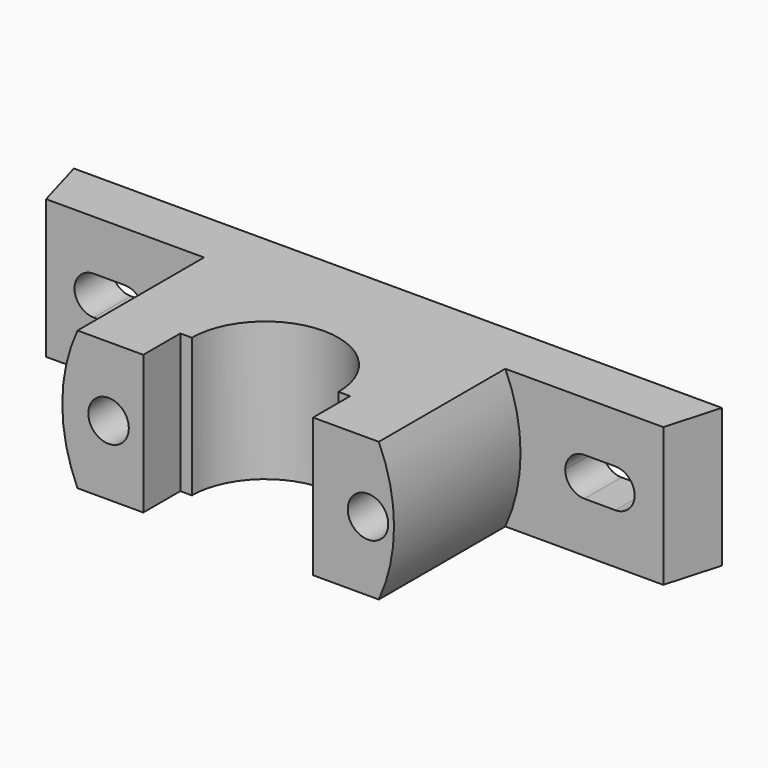
from build123d import *

# Parameters (mm, degrees)
F0_W         = 168
F0_H         = 36
F1_DEPTH     = 14
F3_DEPTH     = 36.001
F5_DEPTH     = 41
F6_R         = 5.25
F7_DEPTH     = 55.001
F8_W         = 20
F8_H         = 20
F9_DEPTH     = 6.5
F10_W        = 67
F10_H        = 20
F11_DEPTH    = 2
F12_T1_DEPTH = 34.1421356237
F14_DEPTH    = 25
F16_DEPTH    = 36.001


# Not quite as in the source:
# - a fillet or chamfer that OpenCascade refuses, or shapes differently, is made with other operations: its cross-section is extruded or revolved along the edge and cut away or added


with BuildPart() as f1:
    # F0 (on Front) → F1 (new body)
    with BuildSketch(Plane.XZ):
        Rectangle(F0_W, F0_H)
    extrude(amount=F1_DEPTH)

    # F2 (on face) → F3 (cut, through all)
    with BuildSketch(Plane(origin=(0, 0, -18), x_dir=(1, 0, 0), z_dir=(0, 0, -1))):
        Polygon((-84, 14), (-84, 0), (-80, 14), align=None)
        Polygon((80, 14), (84, 0), (84, 14), align=None)
    extrude(amount=-F3_DEPTH, mode=Mode.SUBTRACT)

    # F4 (on face) → F5 (join)
    with BuildSketch(Plane.XZ.offset(14)):
        with BuildLine():
            ThreePointArc((39.0512483795, -18), (43, 0), (39.0512483795, 18))
            Line((39.0512483795, 18), (-39.0512483795, 18))
            ThreePointArc((-39.0512483795, 18), (-43, 0), (-39.0512483795, -18))
            Line((-39.0512483795, -18), (39.0512483795, -18))
        make_face()
    extrude(amount=F5_DEPTH)

    # F6 (on face) → F7 (cut, through all)
    with BuildSketch(Plane.XZ.offset(55)):
        with Locations((36.25, 0)):
            Circle(F6_R)
        with Locations((-31, 0)):
            Circle(F6_R)
    extrude(amount=-F7_DEPTH, mode=Mode.SUBTRACT)

    # F8 (on face) → F9 (cut)
    with BuildSketch(Plane(origin=(0, 0, 0), x_dir=(-1, 0, 0), z_dir=(0, 1, 0))):
        with Locations((-36.25, 0)):
            Rectangle(F8_W, F8_H)
        with Locations((31, 0)):
            Rectangle(F8_W, F8_H)
    extrude(amount=-F9_DEPTH, mode=Mode.SUBTRACT)

    # F10 (on face) → F11 (cut)
    with BuildSketch(Plane(origin=(0, 0, 0), x_dir=(-1, 0, 0), z_dir=(0, 1, 0))):
        with Locations((41.5, 0)):
            Rectangle(F10_W, F10_H)
        with Locations((-41.5, 0)):
            Rectangle(F10_W, F10_H)
    extrude(amount=-F11_DEPTH, mode=Mode.SUBTRACT)

    # F12: fillet of radius 3 on 4 edges, made by hand

    # F12_s2 → F12_t1 (join)
    with BuildSketch(Plane.XY.offset(-17.0710678119)):
        with BuildLine():
            ThreePointArc((72.1715728753, -2), (73.9036236828, -1.4494897428), (75, 0))
            Line((75, 0), (75, -2))
            Line((75, -2), (72.1715728753, -2))
        make_face()
        with BuildLine():
            ThreePointArc((10.8284271247, -2), (9.0963763172, -1.4494897428), (8, 0))
            Line((8, 0), (8, -2))
            Line((8, -2), (10.8284271247, -2))
        make_face()
        with BuildLine():
            ThreePointArc((-72.1715728753, -2), (-73.9036236828, -1.4494897428), (-75, 0))
            Line((-75, 0), (-75, -2))
            Line((-75, -2), (-72.1715728753, -2))
        make_face()
        with BuildLine():
            ThreePointArc((-10.8284271247, -2), (-9.0963763172, -1.4494897428), (-8, 0))
            Line((-8, 0), (-8, -2))
            Line((-8, -2), (-10.8284271247, -2))
        make_face()
    extrude(amount=F12_T1_DEPTH)

    # F13 (on face) → F14 (cut)
    with BuildSketch(Plane.XZ.offset(14)):
        with BuildLine():
            ThreePointArc((-67.6350200021, 5), (-72.6350200021, 0), (-67.6350200021, -5))
            Line((-67.6350200021, -5), (-59.6350200021, -5))
            ThreePointArc((-59.6350200021, -5), (-54.6350200021, 0), (-59.6350200021, 5))
            Line((-59.6350200021, 5), (-67.6350200021, 5))
        make_face()
        with BuildLine():
            ThreePointArc((54.5760053992, 0), (56.0404714933, -3.5355339059), (59.5760053992, -5))
            Line((59.5760053992, -5), (67.5760053992, -5))
            ThreePointArc((67.5760053992, -5), (71.1115393052, -3.5355339059), (72.5760053992, 0))
            ThreePointArc((72.5760053992, 0), (71.1115393052, 3.5355339059), (67.5760053992, 5))
            Line((67.5760053992, 5), (59.5760053992, 5))
            ThreePointArc((59.5760053992, 5), (56.0404714933, 3.5355339059), (54.5760053992, 0))
        make_face()
    extrude(amount=-F14_DEPTH, mode=Mode.SUBTRACT)

    # F15 (on face) → F16 (cut, through all)
    with BuildSketch(Plane.XY.offset(18)):
        with BuildLine():
            Line((22, -43), (19, -43))
            ThreePointArc((19, -43), (0, -24), (-19, -43))
            Line((-19, -43), (-22, -43))
            Line((-22, -43), (-22, -55))
            Line((-22, -55), (0, -55))
            Line((0, -55), (22, -55))
            Line((22, -55), (22, -43))
        make_face()
    extrude(amount=-F16_DEPTH, mode=Mode.SUBTRACT)


solid = f1.part
